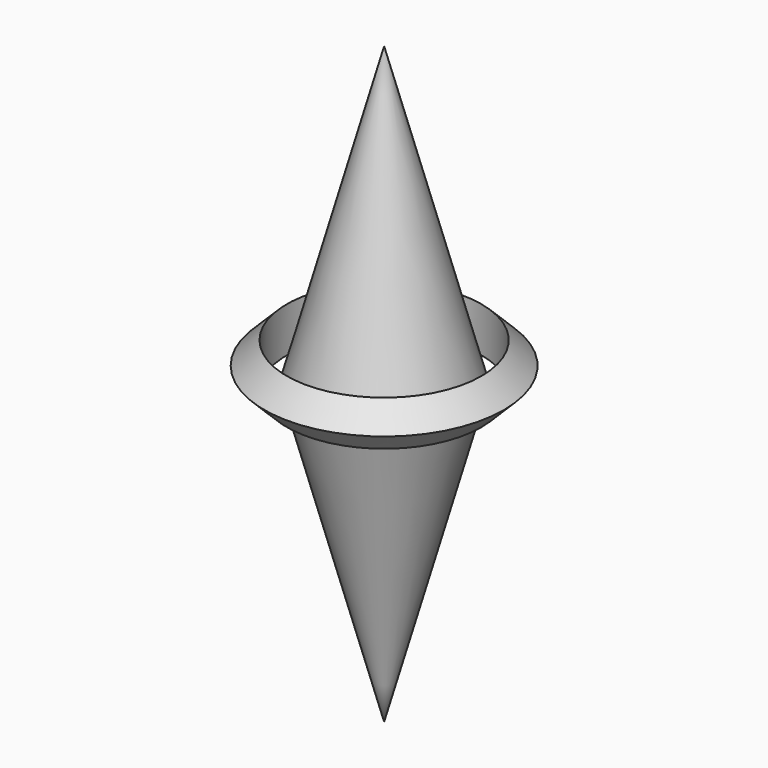
from build123d import *

# Parameters (mm, degrees)
F2_R     = 20.6794561875
F2_R_2   = 16.7980837362
F3_DEPTH = 5


# Not quite as in the source:
# - a fillet or chamfer that OpenCascade refuses, or shapes differently, is made with other operations: its cross-section is extruded or revolved along the edge and cut away or added


with BuildPart() as f1:
    # F0 (on Front) → F1 (revolve)
    with BuildSketch(Plane.XZ):
        Polygon((0, -54.1131310165), (0, 48.5405027866), (-14.0782138333, -2.7863129508), align=None)
    revolve(axis=Axis((0, 0, -2.7863141149), (0, 0, 1)))


with BuildPart() as f3:
    # F2 (on Top) → F3 (new body, symmetric)
    with BuildSketch(Plane.XY):
        Circle(F2_R)
        Circle(F2_R_2, mode=Mode.SUBTRACT)
    extrude(amount=F3_DEPTH, both=True)

    # F4: chamfer of 5 on 2 edges, made by hand

    # F4_s1 → F4_t2 (revolve, cut)
    with BuildSketch(Plane.XZ):
        Polygon((20.6794561875, 0), (15.6794561875, 5), (20.6794561875, 5), align=None)
    revolve(axis=Axis((0, 0, 5), (0, 0, 1)), mode=Mode.SUBTRACT)

    # F4_s3 → F4_t4 (revolve, cut)
    with BuildSketch(Plane.XZ):
        Polygon((20.6794561875, 0), (15.6794561875, -5), (20.6794561875, -5), align=None)
    revolve(axis=Axis((0, 0, -5), (0, 0, 1)), mode=Mode.SUBTRACT)


solid = Compound([f1.part, f3.part])
